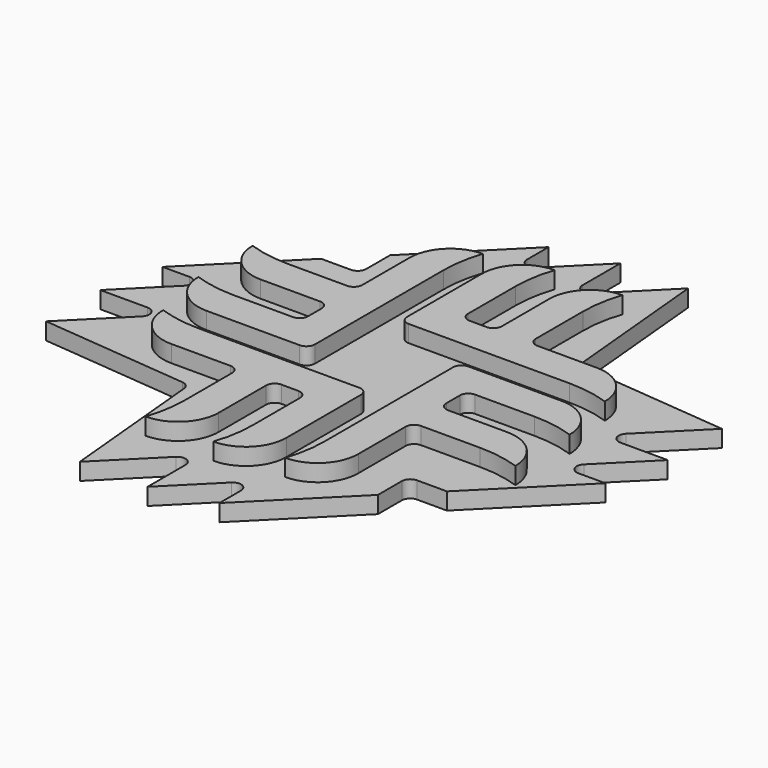
from build123d import *

# Parameters (mm, degrees)
F1_DEPTH = 3.175
F3_DEPTH = 3.175
F4_R     = 1.5875


# Not quite as in the source:
# - a feature names something its author has since deleted; it is built from what else it names


with BuildPart() as f1:
    # F0 (on Top) → F1 (new body)
    with BuildSketch(Plane.XY):
        with BuildLine():
            ThreePointArc((11.7475, 5.08), (10.6249679849, 4.6150320151), (10.16, 3.4925))
            Line((10.16, 3.4925), (10.16, -26.67))
            ThreePointArc((10.16, -26.67), (9.8403252404, -30.5325542067), (8.89, -34.29))
            ThreePointArc((8.89, -34.29), (14.2781536726, -32.0581536726), (16.51, -26.67))
            Line((16.51, -26.67), (16.51, -15.5575))
            ThreePointArc((16.51, -15.5575), (16.9749679849, -14.4349679849), (18.0975, -13.97))
            Line((18.0975, -13.97), (29.21, -13.97))
            ThreePointArc((29.21, -13.97), (33.0725542067, -14.2896747596), (36.83, -15.24))
            ThreePointArc((36.83, -15.24), (34.5981536726, -9.8518463274), (29.21, -7.62))
            Line((29.21, -7.62), (18.0975, -7.62))
            ThreePointArc((18.0975, -7.62), (16.9749679849, -7.1550320151), (16.51, -6.0325))
            Line((16.51, -6.0325), (16.51, -2.8575))
            ThreePointArc((16.51, -2.8575), (16.9749679849, -1.7349679849), (18.0975, -1.27))
            Line((18.0975, -1.27), (29.21, -1.27))
            ThreePointArc((29.21, -1.27), (33.0725542067, -1.5896747596), (36.83, -2.54))
            ThreePointArc((36.83, -2.54), (34.5981536726, 2.8481536726), (29.21, 5.08))
            Line((29.21, 5.08), (11.7475, 5.08))
        make_face()
    extrude(amount=F1_DEPTH)


with BuildPart() as f1b:
    # F0 (on Top) → F1, piece 2 (new body)
    with BuildSketch(Plane.XY):
        with BuildLine():
            ThreePointArc((26.67, 10.16), (30.5325542067, 9.8403252404), (34.29, 8.89))
            ThreePointArc((34.29, 8.89), (32.0581536726, 14.2781536726), (26.67, 16.51))
            Line((26.67, 16.51), (15.5575, 16.51))
            ThreePointArc((15.5575, 16.51), (14.4349679849, 16.9749679849), (13.97, 18.0975))
            Line((13.97, 18.0975), (13.97, 29.21))
            ThreePointArc((13.97, 29.21), (14.2896747596, 33.0725542067), (15.24, 36.83))
            ThreePointArc((15.24, 36.83), (9.8518463274, 34.5981536726), (7.62, 29.21))
            Line((7.62, 29.21), (7.62, 18.0975))
            ThreePointArc((7.62, 18.0975), (7.1550320151, 16.9749679849), (6.0325, 16.51))
            Line((6.0325, 16.51), (2.8575, 16.51))
            ThreePointArc((2.8575, 16.51), (1.7349679849, 16.9749679849), (1.27, 18.0975))
            Line((1.27, 18.0975), (1.27, 29.21))
            ThreePointArc((1.27, 29.21), (1.5896747596, 33.0725542067), (2.54, 36.83))
            ThreePointArc((2.54, 36.83), (-2.8481536726, 34.5981536726), (-5.08, 29.21))
            Line((-5.08, 29.21), (-5.08, 11.7475))
            ThreePointArc((-5.08, 11.7475), (-4.6150320151, 10.6249679849), (-3.4925, 10.16))
            Line((-3.4925, 10.16), (26.67, 10.16))
        make_face()
    extrude(amount=F1_DEPTH)


with BuildPart() as f1c:
    # F0 (on Top) → F1, piece 3 (new body)
    with BuildSketch(Plane.XY):
        with BuildLine():
            ThreePointArc((-10.16, 26.67), (-9.8403252404, 30.5325542067), (-8.89, 34.29))
            ThreePointArc((-8.89, 34.29), (-14.2781536726, 32.0581536726), (-16.51, 26.67))
            Line((-16.51, 26.67), (-16.51, 15.5575))
            ThreePointArc((-16.51, 15.5575), (-16.9749679849, 14.4349679849), (-18.0975, 13.97))
            Line((-18.0975, 13.97), (-29.21, 13.97))
            ThreePointArc((-29.21, 13.97), (-33.0725542067, 14.2896747596), (-36.83, 15.24))
            ThreePointArc((-36.83, 15.24), (-34.5981536726, 9.8518463274), (-29.21, 7.62))
            Line((-29.21, 7.62), (-18.0975, 7.62))
            ThreePointArc((-18.0975, 7.62), (-16.9749679849, 7.1550320151), (-16.51, 6.0325))
            Line((-16.51, 6.0325), (-16.51, 2.8575))
            ThreePointArc((-16.51, 2.8575), (-16.9749679849, 1.7349679849), (-18.0975, 1.27))
            Line((-18.0975, 1.27), (-29.21, 1.27))
            ThreePointArc((-29.21, 1.27), (-33.0725542067, 1.5896747596), (-36.83, 2.54))
            ThreePointArc((-36.83, 2.54), (-34.5981536726, -2.8481536726), (-29.21, -5.08))
            Line((-29.21, -5.08), (-11.7475, -5.08))
            ThreePointArc((-11.7475, -5.08), (-10.6249679849, -4.6150320151), (-10.16, -3.4925))
            Line((-10.16, -3.4925), (-10.16, 26.67))
        make_face()
    extrude(amount=F1_DEPTH)


with BuildPart() as f1d:
    # F0 (on Top) → F1, piece 4 (new body)
    with BuildSketch(Plane.XY):
        with BuildLine():
            ThreePointArc((-26.67, -10.16), (-30.5325542067, -9.8403252404), (-34.29, -8.89))
            ThreePointArc((-34.29, -8.89), (-32.0581536726, -14.2781536726), (-26.67, -16.51))
            Line((-26.67, -16.51), (-15.5575, -16.51))
            ThreePointArc((-15.5575, -16.51), (-14.4349679849, -16.9749679849), (-13.97, -18.0975))
            Line((-13.97, -18.0975), (-13.97, -29.21))
            ThreePointArc((-13.97, -29.21), (-14.2896747596, -33.0725542067), (-15.24, -36.83))
            ThreePointArc((-15.24, -36.83), (-9.8518463274, -34.5981536726), (-7.62, -29.21))
            Line((-7.62, -29.21), (-7.62, -18.0975))
            ThreePointArc((-7.62, -18.0975), (-7.1550320151, -16.9749679849), (-6.0325, -16.51))
            Line((-6.0325, -16.51), (-2.8575, -16.51))
            ThreePointArc((-2.8575, -16.51), (-1.7349679849, -16.9749679849), (-1.27, -18.0975))
            Line((-1.27, -18.0975), (-1.27, -29.21))
            ThreePointArc((-1.27, -29.21), (-1.5896747596, -33.0725542067), (-2.54, -36.83))
            ThreePointArc((-2.54, -36.83), (2.8481536726, -34.5981536726), (5.08, -29.21))
            Line((5.08, -29.21), (5.08, -11.7475))
            ThreePointArc((5.08, -11.7475), (4.6150320151, -10.6249679849), (3.4925, -10.16))
            Line((3.4925, -10.16), (-26.67, -10.16))
        make_face()
    extrude(amount=F1_DEPTH)


with BuildPart() as f3:
    # F2 (on Top) → F3 (new body)
    with BuildSketch(Plane.XY):
        Polygon((6.5305114715, -37.8447175555), (6.5305114715, -46.7347176839), (23.0405122421, -30.2247169133), (23.0405122421, -23.0405122421), (30.2247169133, -23.0405122421), (46.7347176839, -6.5305114715), (37.8447175555, -6.5305114715), (49.2747179408, 4.8994889138), (36.5747179408, 4.8994889138), (49.2747179408, 17.5994889138), (20.3200007064, 20.3200007064), (17.5994889138, 49.2747179408), (4.8994889138, 36.5747179408), (4.8994889138, 49.2747179408), (-6.5305114715, 37.8447175555), (-6.5305114715, 46.7347176839), (-23.0405122421, 30.2247169133), (-23.0405122421, 23.0405122421), (-30.2247169133, 23.0405122421), (-46.7347176839, 6.5305114715), (-37.8447175555, 6.5305114715), (-49.2747179408, -4.8994889138), (-36.5747179408, -4.8994889138), (-49.2747179408, -17.5994889138), (-20.3200007064, -20.3200007064), (-17.5994889138, -49.2747179408), (-4.8994889138, -36.5747179408), (-4.8994889138, -49.2747179408), align=None)
    extrude(amount=-F3_DEPTH)

    # F4
    f4_edges = [f3.edges().sort_by_distance(p)[0] for p in [
        (-37.844718, 6.530511, -1.5875),
        (-36.574718, -4.899489, -1.5875),
        (-23.040512, 23.040512, -1.5875),
        (-6.530511, 37.844718, -1.5875),
        (4.899489, 36.574718, -1.5875),
        (-4.899489, -36.574718, -1.5875),
        (6.530511, -37.844718, -1.5875),
        (23.040512, -23.040512, -1.5875),
        (37.844718, -6.530511, -1.5875),
        (36.574718, 4.899489, -1.5875),
        (20.320001, 20.320001, -1.5875),
        (-20.320001, -20.320001, -1.5875),
    ]]
    fillet(f4_edges, radius=F4_R)


solid = Compound([f1.part, f1b.part, f1c.part, f1d.part, f3.part])
